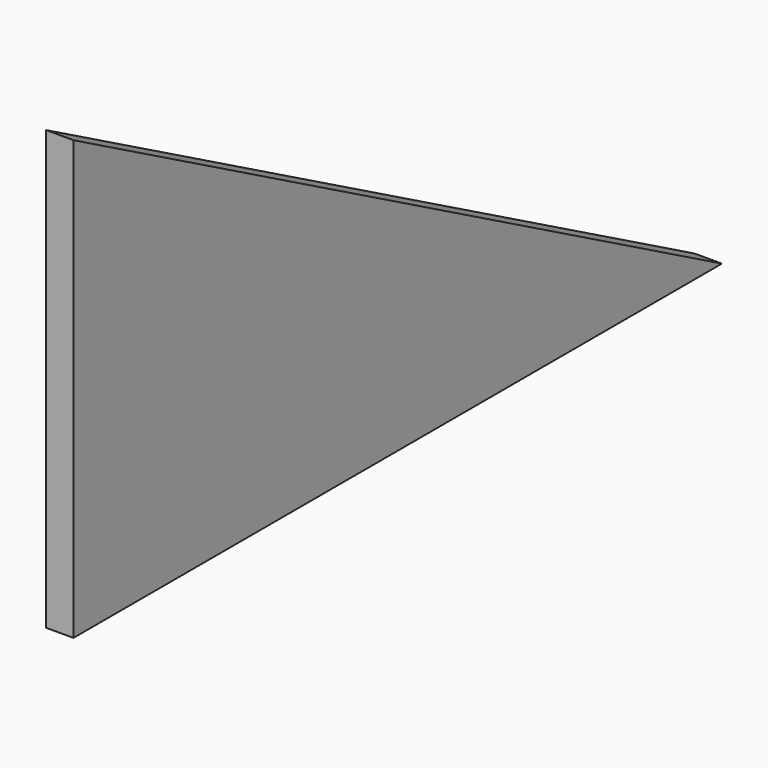
from build123d import *

# Parameters (mm, degrees)
F1_DEPTH = 3.175


# Not quite as in the source:
# - a length typed as a fraction of an inch, garbled in the dataset ("3 / 203.2 mm" for 3/8 in), is restored


with BuildPart() as f1:
    # F0 (on Right) → F1 (new body)
    with BuildSketch(Plane.YZ):
        Polygon((-53.1119635351, 50.8), (-53.1119635351, 0), (40.8680364649, 0), align=None)
    extrude(amount=F1_DEPTH)


solid = f1.part
